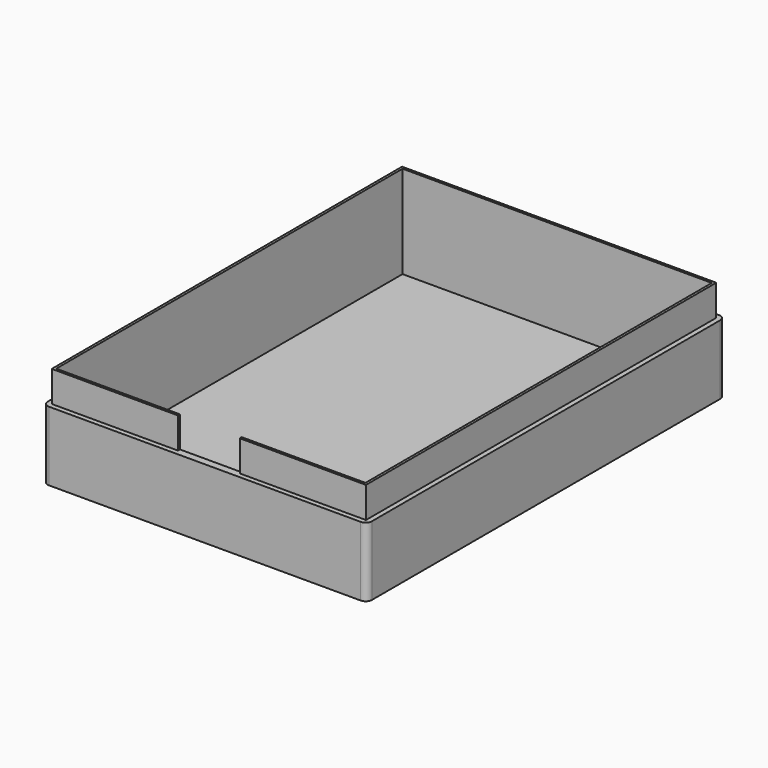
from build123d import *

# Parameters (mm, degrees)
F0_W     = 50
F0_H     = 70
F1_DEPTH = 15
F2_T     = 1.2
F3_W     = 52.4
F3_H     = 72.4
F3_W_2   = 50.8
F3_H_2   = 70.8
F4_DEPTH = 5
F5_R     = 1
F6_W     = 10
F6_H     = 10
F7_DEPTH = 25


with BuildPart() as f1:
    # F0 (on Top) → F1 (new body)
    with BuildSketch(Plane.XY):
        with Locations((25, 35)):
            Rectangle(F0_W, F0_H)
    extrude(amount=F1_DEPTH)

    # F2
    f2_openings = [f1.faces().sort_by_distance(p)[0] for p in [
        (25, 35, 15),
    ]]
    offset(amount=F2_T, openings=f2_openings, kind=Kind.INTERSECTION)

    # F3 (on face) → F4 (cut)
    with BuildSketch(Plane.XY.offset(15)):
        with Locations((25, 35)):
            Rectangle(F3_W, F3_H)
        with Locations((25, 35)):
            Rectangle(F3_W_2, F3_H_2, mode=Mode.SUBTRACT)
    extrude(amount=-F4_DEPTH, mode=Mode.SUBTRACT)

    # F5
    f5_edges = [f1.edges().sort_by_distance(p)[0] for p in [
        (-1.2, 71.2, 4.4),
        (-1.2, -1.2, 4.4),
        (51.2, -1.2, 4.4),
        (51.2, 71.2, 4.4),
    ]]
    fillet(f5_edges, radius=F5_R)

    # F6 (on face) → F7 (cut)
    with BuildSketch(Plane.XZ.offset(1.2)):
        with Locations((25, 15)):
            Rectangle(F6_W, F6_H)
    extrude(amount=-F7_DEPTH, mode=Mode.SUBTRACT)


solid = f1.part
